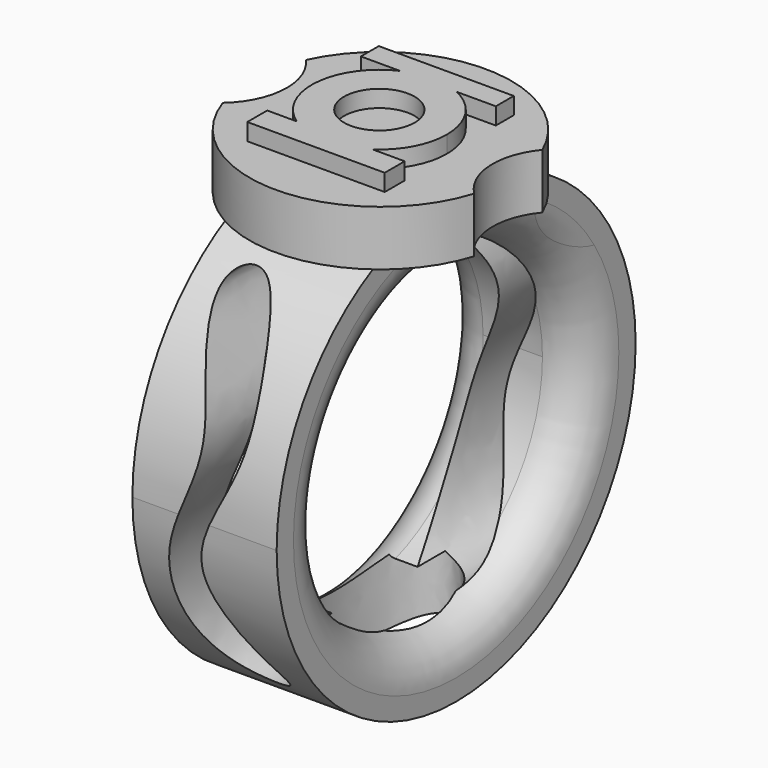
from build123d import *

# Parameters (mm, degrees)
F0_R      = 9.632316
F1_DEPTH  = 8.636
F2_R      = 2.54
F4_R      = 5.942561
F5_DEPTH  = 27.94
F8_R      = 7.842948
F9_DEPTH  = 3.302
F10_R     = 2.111507
F11_DEPTH = 4.318
F13_DEPTH = 45.974
F15_DEPTH = 20.32
F17_DEPTH = 54.864
F19_DEPTH = 19.05


with BuildPart() as f1:
    # F0 (on Right) → F1 (new body)
    with BuildSketch(Plane.YZ):
        with BuildLine():
            ThreePointArc((-4.657582, 21.72097), (-7.67362, -1.892749), (13.427987, 9.126616))
            ThreePointArc((13.427987, 9.126616), (11.047782, 16.759265), (4.750984, 21.686034))
            ThreePointArc((4.750984, 21.686034), (0.035929, 18.802584), (-4.657582, 21.72097))
        make_face()
        with Locations((0, 9.126616)):
            Circle(F0_R, mode=Mode.SUBTRACT)
        with BuildLine():
            ThreePointArc((-4.657582, 21.72097), (0.035929, 18.802584), (4.750984, 21.686034))
            ThreePointArc((4.750984, 21.686034), (0.049861, 22.55451), (-4.657582, 21.72097))
        make_face()
        with BuildLine():
            ThreePointArc((-4.657582, 21.72097), (0.049861, 22.55451), (4.750984, 21.686034))
            ThreePointArc((4.750984, 21.686034), (0.055465, 24.063687), (-4.657582, 21.72097))
        make_face()
    extrude(amount=F1_DEPTH)

    # F2
    f2_edges = [f1.edges().sort_by_distance(p)[0] for p in [
        (8.636, -9.632316, 9.126616),
        (0, -9.632316, 9.126616),
    ]]
    fillet(f2_edges, radius=F2_R)

    # F4 (on Right) → F5 (cut)
    with BuildSketch(Plane.YZ):
        with Locations((11.388008, 21.414585)):
            Circle(F4_R)
    extrude(amount=F5_DEPTH, mode=Mode.SUBTRACT)

    # F6: F1 across plane


with BuildPart() as f1_1:
    add(f1.part)
    add(f1.part.mirror(Plane.XZ))

    # F8 (on offset) → F9 (join)
    with BuildSketch(Plane.XY.offset(21.082)):
        with Locations((4.106977, 0)):
            Circle(F8_R)
    extrude(amount=F9_DEPTH)

    # F10 (on offset) → F11 (join)
    with BuildSketch(Plane.XY.offset(21.082)):
        with BuildLine():
            Line((8.077904, 5.007884), (0, 5.007884))
            Line((0, 5.007884), (0, 3.666291))
            Line((0, 3.666291), (2.344418, 3.666291))
            ThreePointArc((2.344418, 3.666291), (4.038952, 4.038952), (5.733486, 3.666291))
            Line((5.733486, 3.666291), (8.077904, 3.666291))
            Line((8.077904, 3.666291), (8.077904, 5.007884))
        make_face()
        with BuildLine():
            ThreePointArc((5.733486, 3.666291), (4.038952, 4.038952), (2.344418, 3.666291))
            Line((2.344418, 3.666291), (5.733486, 3.666291))
        make_face()
        with BuildLine():
            Line((5.733486, 3.666291), (2.344418, 3.666291))
            ThreePointArc((2.344418, 3.666291), (0.013617, 0.331379), (1.767652, -3.33981))
            Line((1.767652, -3.33981), (6.310251, -3.33981))
            ThreePointArc((6.310251, -3.33981), (7.608742, -1.889373), (8.077904, 0))
            ThreePointArc((8.077904, 0), (7.441691, 2.17589), (5.733486, 3.666291))
        make_face()
        with Locations((4.038952, 0)):
            Circle(F10_R, mode=Mode.SUBTRACT)
        with BuildLine():
            ThreePointArc((6.310251, -3.33981), (4.038952, -4.038952), (1.767652, -3.33981))
            Line((1.767652, -3.33981), (0, -3.33981))
            Line((0, -3.33981), (0, -4.830469))
            Line((0, -4.830469), (8.226969, -4.830469))
            Line((8.226969, -4.830469), (8.226969, -3.33981))
            Line((8.226969, -3.33981), (6.310251, -3.33981))
        make_face()
        with BuildLine():
            Line((6.310251, -3.33981), (1.767652, -3.33981))
            ThreePointArc((1.767652, -3.33981), (4.038952, -4.038952), (6.310251, -3.33981))
        make_face()
    extrude(amount=F11_DEPTH)

    # F12 (on Front) → F13 (cut)
    with BuildSketch(Plane.XZ):
        with BuildLine():
            add(Edge.make_bspline(
                [(1.917409, 19.37164), (1.574813, 18.182006), (5.617537, 13.038047), (1.16523, 7.576133), (2.518197, -0.802501), (8.69957, -0.671948), (1.781667, 6.845731), (8.008673, 12.629879), (4.952165, 20.746919), (2.120158, 20.075669), (1.917409, 19.37164)],
                knots=[0, 0, 0, 0, 0.131665, 0.269486, 0.411759, 0.500255, 0.638086, 0.782487, 0.92208, 1, 1, 1, 1], degree=3))
        make_face()
    extrude(amount=-F13_DEPTH, mode=Mode.SUBTRACT)

    # F14 (on Front) → F15 (cut)
    with BuildSketch(Plane.XZ):
        with BuildLine():
            add(Edge.make_bspline(
                [(1.791432, 19.315292), (1.448836, 18.125658), (5.49156, 12.981699), (1.039253, 7.519786), (2.39222, -0.858848), (8.573593, -0.728296), (1.65569, 6.789383), (7.882696, 12.573531), (4.826188, 20.690571), (1.994181, 20.019321), (1.791432, 19.315292)],
                knots=[0, 0, 0, 0, 0.131665, 0.269486, 0.411759, 0.500255, 0.638086, 0.782487, 0.92208, 1, 1, 1, 1], degree=3))
        make_face()
    extrude(amount=F15_DEPTH, mode=Mode.SUBTRACT)

    # F16 (on Top) → F17 (cut)
    with BuildSketch(Plane.XY):
        with BuildLine():
            ThreePointArc((14.602585, -3.498536), (21.26904, 0.408039), (14.754695, 4.563308))
            ThreePointArc((14.754695, 4.563308), (10.38637, 0.613372), (14.602585, -3.498536))
        make_face()
        with BuildLine():
            ThreePointArc((-6.621435, 4.563308), (-12.255805, 0.263129), (-6.248515, -3.498536))
            ThreePointArc((-6.248515, -3.498536), (-1.938323, 0.74039), (-6.621435, 4.563308))
        make_face()
    extrude(amount=F17_DEPTH, mode=Mode.SUBTRACT)

    # F18 (on Top) → F19 (cut)
    with BuildSketch(Plane.XY):
        with BuildLine():
            add(Edge.make_bspline(
                [(4.173733, -5.168469), (8.916121, -5.168469), (6.544927, 2.584234), (4.173733, 10.336937), (1.802538, 2.584234), (-0.568656, -5.168469), (4.173733, -5.168469)],
                knots=[0, 0, 0, 2.094395, 2.094395, 4.18879, 4.18879, 6.283185, 6.283185, 6.283185], degree=2, weights=[1, 0.5, 1, 0.5, 1, 0.5, 1]))
        make_face()
    extrude(amount=-F19_DEPTH, mode=Mode.SUBTRACT)


solid = f1_1.part
